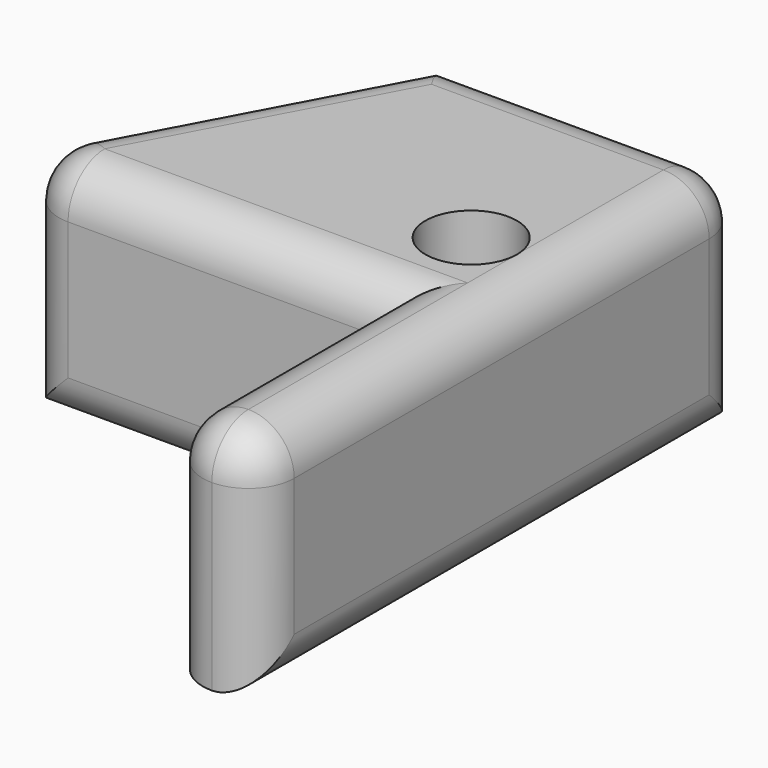
from build123d import *

# Parameters (mm, degrees)
F1_DEPTH = 15
F2_R     = 3
F3_DEPTH = 25
F4_R     = 2.99999


# Not quite as in the source:
# - a fillet or chamfer is up to 0.001 mm smaller than in the source, because OpenCascade refuses the exact size


with BuildPart() as f1:
    # F0 (on Top) → F1 (new body)
    with BuildSketch(Plane.XY):
        Polygon((-6, 0), (0, 0), (0, 40), (-20, 40), (-31.8061554718, 17.9633329885), (-6, 17.9633329885), align=None)
    extrude(amount=F1_DEPTH)

    # F2 (on face) → F3 (cut)
    with BuildSketch(Plane.XY.offset(15)):
        with Locations((-6, 25)):
            Circle(F2_R)
    extrude(amount=-F3_DEPTH, mode=Mode.SUBTRACT)

    # F4 (radius 3 in the source; OpenCascade refuses exactly that, so slightly less here)
    f4_edges = [f1.edges().sort_by_distance(p)[0] for p in [
        (0, 20, 15),
        (-6, 8.981666, 15),
        (-18.903078, 17.963333, 15),
        (-25.903078, 28.981666, 15),
        (-10, 40, 15),
        (0, 40, 7.5),
        (-3, 0, 15),
        (0, 0, 7.5),
        (0, 20, 0),
        (-18.903078, 17.963333, 0),
        (-31.806155, 17.963333, 7.5),
        (-6, 0, 7.5),
    ]]
    fillet(f4_edges, radius=F4_R)


solid = f1.part
